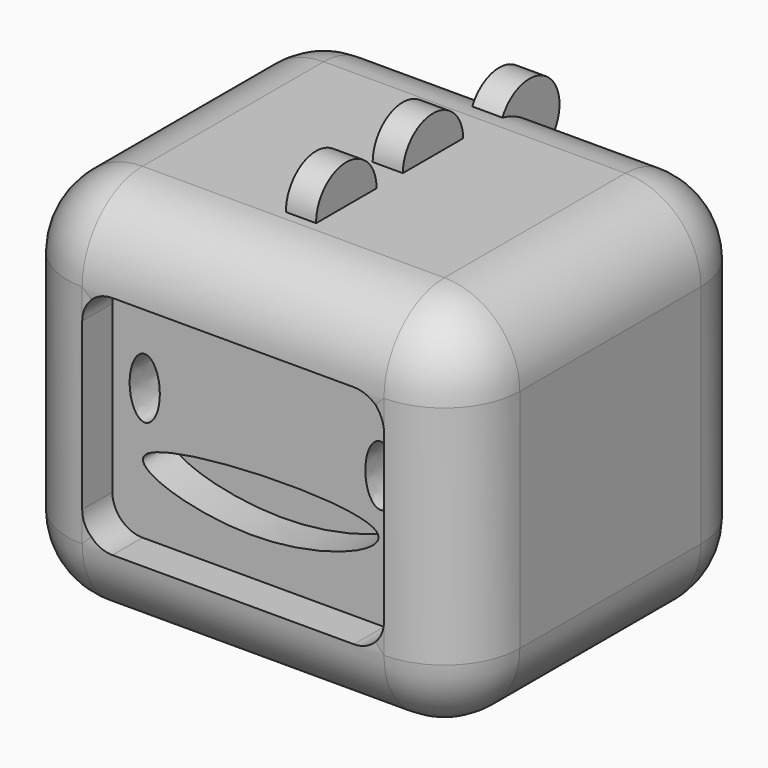
from build123d import *

# Parameters (mm, degrees)
F1_DEPTH       = 63.5
F2_R           = 12.7
F3_DEPTH       = 6.35
F4_T4_DEPTH    = 19.05
F4_S5_R        = 12.7
F4_T6_DEPTH    = 12
F4_S7_R        = 12.7
F4_T8_DEPTH    = 12
F4_T12_DEPTH   = 19.05
F4_S13_R       = 12.7
F4_T14_DEPTH   = 12
F4_S15_R       = 12.7
F4_T16_DEPTH   = 12
F4_T20_DEPTH   = 19.05
F4_S21_R       = 12.7
F4_T22_DEPTH   = 12
F4_S23_R       = 12.7
F4_T24_DEPTH   = 12
F4_T28_DEPTH   = 31.75
F4_T33_DEPTH   = 19.05
F4_S34_R       = 12.7
F4_T35_DEPTH   = 12
F4_S36_R       = 12.7
F4_T37_DEPTH   = 12
F4_T41_DEPTH   = 19.05
F4_S42_R       = 12.7
F4_T43_DEPTH   = 12
F4_S44_R       = 12.7
F4_T45_DEPTH   = 12
F4_T49_DEPTH   = 19.05
F4_S50_R       = 12.7
F4_T51_DEPTH   = 12
F4_S52_R       = 12.7
F4_T53_DEPTH   = 12
F4_T57_DEPTH   = 31.75
F4_T62_DEPTH   = 19.05
F4_S63_R       = 12.7
F4_T64_DEPTH   = 12
F4_S65_R       = 12.7
F4_T66_DEPTH   = 12
F4_T70_DEPTH   = 19.05
F4_S71_R       = 12.7
F4_T72_DEPTH   = 12
F4_S73_R       = 12.7
F4_T74_DEPTH   = 12
F4_T78_DEPTH   = 19.05
F4_S79_R       = 12.7
F4_T80_DEPTH   = 12
F4_S81_R       = 12.7
F4_T82_DEPTH   = 12
F4_T86_DEPTH   = 31.75
F4_T91_DEPTH   = 19.05
F4_S92_R       = 12.7
F4_T93_DEPTH   = 12
F4_S94_R       = 12.7
F4_T95_DEPTH   = 12
F4_T99_DEPTH   = 19.05
F4_S100_R      = 12.7
F4_T101_DEPTH  = 12
F4_S102_R      = 12.7
F4_T103_DEPTH  = 12
F4_T107_DEPTH  = 19.05
F4_S108_R      = 12.7
F4_T109_DEPTH  = 12
F4_S110_R      = 12.7
F4_T111_DEPTH  = 12
F4_T115_DEPTH  = 31.75
F7_DEPTH       = 6.35
F9_DEPTH       = 6.35
F10_R          = 6.35
F11_DEPTH      = 2.54
F11_DEPTH_BACK = 2.54


# Not quite as in the source:
# - a fillet or chamfer that OpenCascade refuses, or shapes differently, is made with other operations: its cross-section is extruded or revolved along the edge and cut away or added


with BuildPart() as f1:
    # F0 (on Top) → F1 (new body)
    with BuildSketch(Plane.XY):
        with BuildLine():
            ThreePointArc((38.1, 19.05), (34.3802561211, 28.0302561211), (25.4, 31.75))
            Line((25.4, 31.75), (-25.4, 31.75))
            ThreePointArc((-25.4, 31.75), (-34.3802561211, 28.0302561211), (-38.1, 19.05))
            Line((-38.1, 19.05), (-38.1, -19.05))
            ThreePointArc((-38.1, -19.05), (-34.3802561211, -28.0302561211), (-25.4, -31.75))
            Line((-25.4, -31.75), (25.4, -31.75))
            ThreePointArc((25.4, -31.75), (34.3802561211, -28.0302561211), (38.1, -19.05))
            Line((38.1, -19.05), (38.1, 19.05))
        make_face()
    extrude(amount=F1_DEPTH)

    # F2
    f2_edges = [f1.edges().sort_by_distance(p)[0] for p in [
        (34.380256, 28.030256, 63.5),
        (0, 31.75, 63.5),
        (-34.380256, 28.030256, 63.5),
        (-38.1, 0, 63.5),
        (-34.380256, -28.030256, 63.5),
        (0, -31.75, 63.5),
        (34.380256, -28.030256, 63.5),
        (38.1, 0, 63.5),
        (34.380256, 28.030256, 0),
        (0, 31.75, 0),
        (-34.380256, 28.030256, 0),
        (-38.1, 0, 0),
        (-34.380256, -28.030256, 0),
        (0, -31.75, 0),
        (34.380256, -28.030256, 0),
        (38.1, 0, 0),
    ]]
    fillet(f2_edges, radius=F2_R)

    # F3 (cut): a face of the model
    f3_faces = [f1.faces().sort_by_distance(p)[0] for p in [
        (0, -31.75, 31.75),
    ]]
    extrude(f3_faces, amount=-F3_DEPTH, mode=Mode.SUBTRACT)

    # F4: fillet of radius 5.08 on 4 edges, made by hand


with BuildPart() as f4_tool2:
    # F4_s3 → F4_t4 (new body)
    with BuildSketch(Plane.XZ.offset(44.45)):
        with BuildLine():
            ThreePointArc((25.4, 17.78), (23.9121024484, 14.1878975516), (20.32, 12.7))
            Line((20.32, 12.7), (25.4, 12.7))
            Line((25.4, 12.7), (25.4, 17.78))
        make_face()
    extrude(amount=-F4_T4_DEPTH)

    # F4_s5 → F4_t6 (cut, symmetric)
    with BuildSketch(Plane.XY.offset(15.2)):
        with Locations((25.4, -19.05)):
            Circle(F4_S5_R)
    extrude(amount=F4_T6_DEPTH, both=True, mode=Mode.SUBTRACT)

    # F4_s7 → F4_t8 (intersect, symmetric)
    with BuildSketch(Plane.YZ.offset(22.9)):
        with Locations((-19.05, 12.7)):
            Circle(F4_S7_R)
    extrude(amount=F4_T8_DEPTH, both=True, mode=Mode.INTERSECT)


with BuildPart() as f1_1:
    add(f1.part)

    # F4_t1: union F4_tool2
    add(f4_tool2.part)


with BuildPart() as f4_tool10:
    # F4_s11 → F4_t12 (new body)
    with BuildSketch(Plane.XZ.offset(44.45)):
        with BuildLine():
            ThreePointArc((25.4, 17.78), (23.9121024484, 14.1878975516), (20.32, 12.7))
            Line((20.32, 12.7), (25.4, 12.7))
            Line((25.4, 12.7), (25.4, 17.78))
        make_face()
    extrude(amount=-F4_T12_DEPTH)

    # F4_s13 → F4_t14 (intersect, symmetric)
    with BuildSketch(Plane.XY.offset(15.2)):
        with Locations((25.4, -19.05)):
            Circle(F4_S13_R)
    extrude(amount=F4_T14_DEPTH, both=True, mode=Mode.INTERSECT)

    # F4_s15 → F4_t16 (cut, symmetric)
    with BuildSketch(Plane.YZ.offset(22.9)):
        with Locations((-19.05, 12.7)):
            Circle(F4_S15_R)
    extrude(amount=F4_T16_DEPTH, both=True, mode=Mode.SUBTRACT)


with BuildPart() as f1_2:
    add(f1_1.part)

    # F4_t9: union F4_tool10
    add(f4_tool10.part)


with BuildPart() as f4_tool18:
    # F4_s19 → F4_t20 (new body)
    with BuildSketch(Plane.XZ.offset(44.45)):
        with BuildLine():
            ThreePointArc((25.4, 17.78), (23.9121024484, 14.1878975516), (20.32, 12.7))
            Line((20.32, 12.7), (25.4, 12.7))
            Line((25.4, 12.7), (25.4, 17.78))
        make_face()
    extrude(amount=-F4_T20_DEPTH)

    # F4_s21 → F4_t22 (intersect, symmetric)
    with BuildSketch(Plane.XY.offset(15.2)):
        with Locations((25.4, -19.05)):
            Circle(F4_S21_R)
    extrude(amount=F4_T22_DEPTH, both=True, mode=Mode.INTERSECT)

    # F4_s23 → F4_t24 (intersect, symmetric)
    with BuildSketch(Plane.YZ.offset(22.9)):
        with Locations((-19.05, 12.7)):
            Circle(F4_S23_R)
    extrude(amount=F4_T24_DEPTH, both=True, mode=Mode.INTERSECT)


with BuildPart() as f1_3:
    add(f1_2.part)

    # F4_t17: union F4_tool18
    add(f4_tool18.part)


with BuildPart() as f4_tool26:
    # F4_s27 → F4_t28 (new body)
    with BuildSketch(Plane.XZ.offset(44.45)):
        with BuildLine():
            ThreePointArc((25.4, 17.78), (23.9121024484, 14.1878975516), (20.32, 12.7))
            Line((20.32, 12.7), (25.4, 12.7))
            Line((25.4, 12.7), (25.4, 17.78))
        make_face()
    extrude(amount=-F4_T28_DEPTH)

    split(bisect_by=Plane.XZ.offset(25.4), keep=Keep.BOTTOM)


with BuildPart() as f1_4:
    add(f1_3.part)

    # F4_t25: union F4_tool26
    add(f4_tool26.part)


with BuildPart() as f4_tool31:
    # F4_s32 → F4_t33 (new body)
    with BuildSketch(Plane.XZ.offset(44.45)):
        with BuildLine():
            ThreePointArc((25.4, 45.72), (23.9121024484, 49.3121024484), (20.32, 50.8))
            Line((20.32, 50.8), (25.4, 50.8))
            Line((25.4, 50.8), (25.4, 45.72))
        make_face()
    extrude(amount=-F4_T33_DEPTH)

    # F4_s34 → F4_t35 (cut, symmetric)
    with BuildSketch(Plane.XY.offset(48.3)):
        with Locations((25.4, -19.05)):
            Circle(F4_S34_R)
    extrude(amount=F4_T35_DEPTH, both=True, mode=Mode.SUBTRACT)

    # F4_s36 → F4_t37 (intersect, symmetric)
    with BuildSketch(Plane.YZ.offset(22.9)):
        with Locations((-19.05, 50.8)):
            Circle(F4_S36_R)
    extrude(amount=F4_T37_DEPTH, both=True, mode=Mode.INTERSECT)


with BuildPart() as f1_5:
    add(f1_4.part)

    # F4_t30: union F4_tool31
    add(f4_tool31.part)


with BuildPart() as f4_tool39:
    # F4_s40 → F4_t41 (new body)
    with BuildSketch(Plane.XZ.offset(44.45)):
        with BuildLine():
            ThreePointArc((25.4, 45.72), (23.9121024484, 49.3121024484), (20.32, 50.8))
            Line((20.32, 50.8), (25.4, 50.8))
            Line((25.4, 50.8), (25.4, 45.72))
        make_face()
    extrude(amount=-F4_T41_DEPTH)

    # F4_s42 → F4_t43 (intersect, symmetric)
    with BuildSketch(Plane.XY.offset(48.3)):
        with Locations((25.4, -19.05)):
            Circle(F4_S42_R)
    extrude(amount=F4_T43_DEPTH, both=True, mode=Mode.INTERSECT)

    # F4_s44 → F4_t45 (cut, symmetric)
    with BuildSketch(Plane.YZ.offset(22.9)):
        with Locations((-19.05, 50.8)):
            Circle(F4_S44_R)
    extrude(amount=F4_T45_DEPTH, both=True, mode=Mode.SUBTRACT)


with BuildPart() as f1_6:
    add(f1_5.part)

    # F4_t38: union F4_tool39
    add(f4_tool39.part)


with BuildPart() as f4_tool47:
    # F4_s48 → F4_t49 (new body)
    with BuildSketch(Plane.XZ.offset(44.45)):
        with BuildLine():
            ThreePointArc((25.4, 45.72), (23.9121024484, 49.3121024484), (20.32, 50.8))
            Line((20.32, 50.8), (25.4, 50.8))
            Line((25.4, 50.8), (25.4, 45.72))
        make_face()
    extrude(amount=-F4_T49_DEPTH)

    # F4_s50 → F4_t51 (intersect, symmetric)
    with BuildSketch(Plane.XY.offset(48.3)):
        with Locations((25.4, -19.05)):
            Circle(F4_S50_R)
    extrude(amount=F4_T51_DEPTH, both=True, mode=Mode.INTERSECT)

    # F4_s52 → F4_t53 (intersect, symmetric)
    with BuildSketch(Plane.YZ.offset(22.9)):
        with Locations((-19.05, 50.8)):
            Circle(F4_S52_R)
    extrude(amount=F4_T53_DEPTH, both=True, mode=Mode.INTERSECT)


with BuildPart() as f1_7:
    add(f1_6.part)

    # F4_t46: union F4_tool47
    add(f4_tool47.part)


with BuildPart() as f4_tool55:
    # F4_s56 → F4_t57 (new body)
    with BuildSketch(Plane.XZ.offset(44.45)):
        with BuildLine():
            ThreePointArc((25.4, 45.72), (23.9121024484, 49.3121024484), (20.32, 50.8))
            Line((20.32, 50.8), (25.4, 50.8))
            Line((25.4, 50.8), (25.4, 45.72))
        make_face()
    extrude(amount=-F4_T57_DEPTH)

    split(bisect_by=Plane.XZ.offset(25.4), keep=Keep.BOTTOM)


with BuildPart() as f1_8:
    add(f1_7.part)

    # F4_t54: union F4_tool55
    add(f4_tool55.part)


with BuildPart() as f4_tool60:
    # F4_s61 → F4_t62 (new body)
    with BuildSketch(Plane.XZ.offset(44.45)):
        with BuildLine():
            ThreePointArc((-20.32, 12.7), (-23.9121024484, 14.1878975516), (-25.4, 17.78))
            Line((-25.4, 17.78), (-25.4, 12.7))
            Line((-25.4, 12.7), (-20.32, 12.7))
        make_face()
    extrude(amount=-F4_T62_DEPTH)

    # F4_s63 → F4_t64 (cut, symmetric)
    with BuildSketch(Plane.YZ.offset(-22.9)):
        with Locations((-19.05, 12.7)):
            Circle(F4_S63_R)
    extrude(amount=F4_T64_DEPTH, both=True, mode=Mode.SUBTRACT)

    # F4_s65 → F4_t66 (intersect, symmetric)
    with BuildSketch(Plane.XY.offset(15.2)):
        with Locations((-25.4, -19.05)):
            Circle(F4_S65_R)
    extrude(amount=F4_T66_DEPTH, both=True, mode=Mode.INTERSECT)


with BuildPart() as f1_9:
    add(f1_8.part)

    # F4_t59: union F4_tool60
    add(f4_tool60.part)


with BuildPart() as f4_tool68:
    # F4_s69 → F4_t70 (new body)
    with BuildSketch(Plane.XZ.offset(44.45)):
        with BuildLine():
            ThreePointArc((-20.32, 12.7), (-23.9121024484, 14.1878975516), (-25.4, 17.78))
            Line((-25.4, 17.78), (-25.4, 12.7))
            Line((-25.4, 12.7), (-20.32, 12.7))
        make_face()
    extrude(amount=-F4_T70_DEPTH)

    # F4_s71 → F4_t72 (intersect, symmetric)
    with BuildSketch(Plane.YZ.offset(-22.9)):
        with Locations((-19.05, 12.7)):
            Circle(F4_S71_R)
    extrude(amount=F4_T72_DEPTH, both=True, mode=Mode.INTERSECT)

    # F4_s73 → F4_t74 (cut, symmetric)
    with BuildSketch(Plane.XY.offset(15.2)):
        with Locations((-25.4, -19.05)):
            Circle(F4_S73_R)
    extrude(amount=F4_T74_DEPTH, both=True, mode=Mode.SUBTRACT)


with BuildPart() as f1_10:
    add(f1_9.part)

    # F4_t67: union F4_tool68
    add(f4_tool68.part)


with BuildPart() as f4_tool76:
    # F4_s77 → F4_t78 (new body)
    with BuildSketch(Plane.XZ.offset(44.45)):
        with BuildLine():
            ThreePointArc((-20.32, 12.7), (-23.9121024484, 14.1878975516), (-25.4, 17.78))
            Line((-25.4, 17.78), (-25.4, 12.7))
            Line((-25.4, 12.7), (-20.32, 12.7))
        make_face()
    extrude(amount=-F4_T78_DEPTH)

    # F4_s79 → F4_t80 (intersect, symmetric)
    with BuildSketch(Plane.YZ.offset(-22.9)):
        with Locations((-19.05, 12.7)):
            Circle(F4_S79_R)
    extrude(amount=F4_T80_DEPTH, both=True, mode=Mode.INTERSECT)

    # F4_s81 → F4_t82 (intersect, symmetric)
    with BuildSketch(Plane.XY.offset(15.2)):
        with Locations((-25.4, -19.05)):
            Circle(F4_S81_R)
    extrude(amount=F4_T82_DEPTH, both=True, mode=Mode.INTERSECT)


with BuildPart() as f1_11:
    add(f1_10.part)

    # F4_t75: union F4_tool76
    add(f4_tool76.part)


with BuildPart() as f4_tool84:
    # F4_s85 → F4_t86 (new body)
    with BuildSketch(Plane.XZ.offset(44.45)):
        with BuildLine():
            ThreePointArc((-20.32, 12.7), (-23.9121024484, 14.1878975516), (-25.4, 17.78))
            Line((-25.4, 17.78), (-25.4, 12.7))
            Line((-25.4, 12.7), (-20.32, 12.7))
        make_face()
    extrude(amount=-F4_T86_DEPTH)

    split(bisect_by=Plane.XZ.offset(25.4), keep=Keep.BOTTOM)


with BuildPart() as f1_12:
    add(f1_11.part)

    # F4_t83: union F4_tool84
    add(f4_tool84.part)


with BuildPart() as f4_tool89:
    # F4_s90 → F4_t91 (new body)
    with BuildSketch(Plane.XZ.offset(44.45)):
        with BuildLine():
            ThreePointArc((-20.32, 50.8), (-23.9121024484, 49.3121024484), (-25.4, 45.72))
            Line((-25.4, 45.72), (-25.4, 50.8))
            Line((-25.4, 50.8), (-20.32, 50.8))
        make_face()
    extrude(amount=-F4_T91_DEPTH)

    # F4_s92 → F4_t93 (cut, symmetric)
    with BuildSketch(Plane.YZ.offset(-22.9)):
        with Locations((-19.05, 50.8)):
            Circle(F4_S92_R)
    extrude(amount=F4_T93_DEPTH, both=True, mode=Mode.SUBTRACT)

    # F4_s94 → F4_t95 (intersect, symmetric)
    with BuildSketch(Plane.XY.offset(48.3)):
        with Locations((-25.4, -19.05)):
            Circle(F4_S94_R)
    extrude(amount=F4_T95_DEPTH, both=True, mode=Mode.INTERSECT)


with BuildPart() as f1_13:
    add(f1_12.part)

    # F4_t88: union F4_tool89
    add(f4_tool89.part)


with BuildPart() as f4_tool97:
    # F4_s98 → F4_t99 (new body)
    with BuildSketch(Plane.XZ.offset(44.45)):
        with BuildLine():
            ThreePointArc((-20.32, 50.8), (-23.9121024484, 49.3121024484), (-25.4, 45.72))
            Line((-25.4, 45.72), (-25.4, 50.8))
            Line((-25.4, 50.8), (-20.32, 50.8))
        make_face()
    extrude(amount=-F4_T99_DEPTH)

    # F4_s100 → F4_t101 (intersect, symmetric)
    with BuildSketch(Plane.YZ.offset(-22.9)):
        with Locations((-19.05, 50.8)):
            Circle(F4_S100_R)
    extrude(amount=F4_T101_DEPTH, both=True, mode=Mode.INTERSECT)

    # F4_s102 → F4_t103 (cut, symmetric)
    with BuildSketch(Plane.XY.offset(48.3)):
        with Locations((-25.4, -19.05)):
            Circle(F4_S102_R)
    extrude(amount=F4_T103_DEPTH, both=True, mode=Mode.SUBTRACT)


with BuildPart() as f1_14:
    add(f1_13.part)

    # F4_t96: union F4_tool97
    add(f4_tool97.part)


with BuildPart() as f4_tool105:
    # F4_s106 → F4_t107 (new body)
    with BuildSketch(Plane.XZ.offset(44.45)):
        with BuildLine():
            ThreePointArc((-20.32, 50.8), (-23.9121024484, 49.3121024484), (-25.4, 45.72))
            Line((-25.4, 45.72), (-25.4, 50.8))
            Line((-25.4, 50.8), (-20.32, 50.8))
        make_face()
    extrude(amount=-F4_T107_DEPTH)

    # F4_s108 → F4_t109 (intersect, symmetric)
    with BuildSketch(Plane.YZ.offset(-22.9)):
        with Locations((-19.05, 50.8)):
            Circle(F4_S108_R)
    extrude(amount=F4_T109_DEPTH, both=True, mode=Mode.INTERSECT)

    # F4_s110 → F4_t111 (intersect, symmetric)
    with BuildSketch(Plane.XY.offset(48.3)):
        with Locations((-25.4, -19.05)):
            Circle(F4_S110_R)
    extrude(amount=F4_T111_DEPTH, both=True, mode=Mode.INTERSECT)


with BuildPart() as f1_15:
    add(f1_14.part)

    # F4_t104: union F4_tool105
    add(f4_tool105.part)


with BuildPart() as f4_tool113:
    # F4_s114 → F4_t115 (new body)
    with BuildSketch(Plane.XZ.offset(44.45)):
        with BuildLine():
            ThreePointArc((-20.32, 50.8), (-23.9121024484, 49.3121024484), (-25.4, 45.72))
            Line((-25.4, 45.72), (-25.4, 50.8))
            Line((-25.4, 50.8), (-20.32, 50.8))
        make_face()
    extrude(amount=-F4_T115_DEPTH)

    split(bisect_by=Plane.XZ.offset(25.4), keep=Keep.BOTTOM)


with BuildPart() as f1_16:
    add(f1_15.part)

    # F4_t112: union F4_tool113
    add(f4_tool113.part)

    # F6 (on offset) → F7 (cut)
    with BuildSketch(Plane.XZ.offset(25.4)):
        with BuildLine():
            add(Edge.make_bspline(
                [(-19.9538823217, 40.0411081183), (-24.3532913729, 40.0411081183), (-22.1535868473, 32.4211081183), (-19.9538823217, 24.8011081183), (-17.7541777961, 32.4211081183), (-15.5544732705, 40.0411081183), (-19.9538823217, 40.0411081183)],
                knots=[0, 0, 0, 2.0943951024, 2.0943951024, 4.1887902048, 4.1887902048, 6.2831853072, 6.2831853072, 6.2831853072], degree=2, weights=[1, 0.5, 1, 0.5, 1, 0.5, 1]))
        make_face()
        with BuildLine():
            add(Edge.make_bspline(
                [(19.7207042576, 39.9870246475), (15.3212952063, 39.9870246475), (17.5209997319, 32.3670246475), (19.7207042576, 24.7470246475), (21.9204087832, 32.3670246475), (24.1201133088, 39.9870246475), (19.7207042576, 39.9870246475)],
                knots=[0, 0, 0, 2.0943951024, 2.0943951024, 4.1887902048, 4.1887902048, 6.2831853072, 6.2831853072, 6.2831853072], degree=2, weights=[1, 0.5, 1, 0.5, 1, 0.5, 1]))
        make_face()
    extrude(amount=-F7_DEPTH, mode=Mode.SUBTRACT)

    # F8 (on offset) → F9 (cut)
    with BuildSketch(Plane.XZ.offset(25.4)):
        with BuildLine():
            add(Edge.make_bspline(
                [(-19.8178328574, 25.164861232), (-22.6623498561, 22.5631797606), (0.1459036803, 14.7938469787), (36.8441903107, 30.6531948363), (-15.9304937435, 28.7203394206), (-19.8178328574, 25.164861232)],
                knots=[0, 0, 0, 0, 0.297963223, 0.5928011358, 1, 1, 1, 1], degree=3))
        make_face()
    extrude(amount=-F9_DEPTH, mode=Mode.SUBTRACT)

    # F10 (on Right) → F11 (join, two sides)
    with BuildSketch(Plane.YZ) as f11_sk:
        with Locations((-11.1081842333, 63.6173412204)):
            Circle(F10_R)
        with Locations((7.134210784, 63.4367242455)):
            Circle(F10_R)
        with Locations((27.4023022503, 60.3210888803)):
            Circle(F10_R)
        with Locations((31.947221607, 41.8740585446)):
            Circle(F10_R)
        with Locations((31.6798724234, 24.2290720344)):
            Circle(F10_R)
    extrude(amount=F11_DEPTH)
    extrude(f11_sk.sketch, amount=-F11_DEPTH_BACK)


solid = f1_16.part
